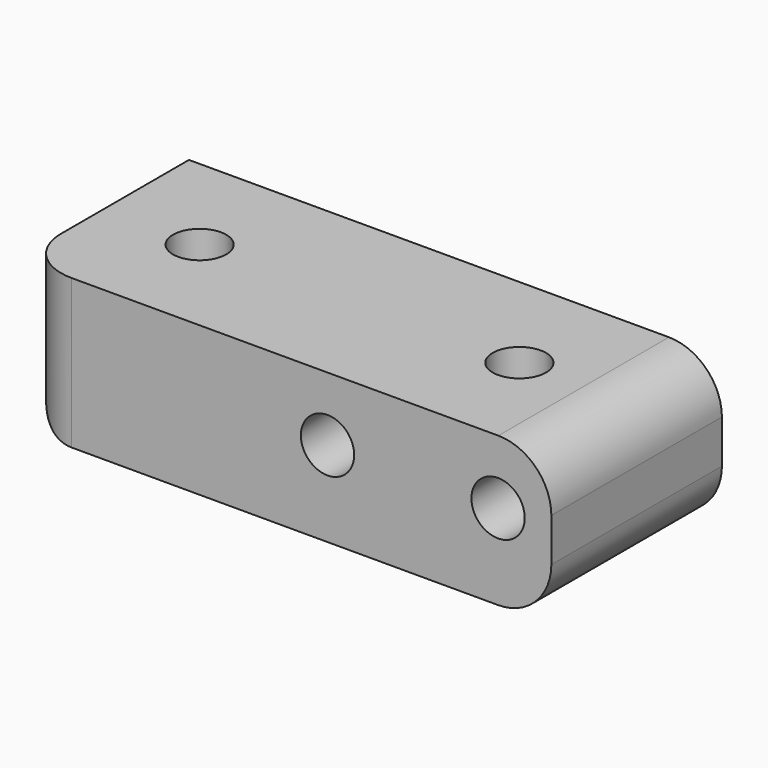
from build123d import *

# Parameters (mm, degrees)
F0_W        = 20
F0_H        = 14
F1_DEPTH    = 25
F3_D        = 5
F5_D        = 5
F6_T1_DEPTH = 44.999500005
F7_T1_DEPTH = 34.0317226184


# Not quite as in the source:
# - a fillet or chamfer that OpenCascade refuses, or shapes differently, is made with other operations: its cross-section is extruded or revolved along the edge and cut away or added


with BuildPart() as f1:
    # F0 (on Right) → F1 (new body, symmetric)
    with BuildSketch(Plane.YZ):
        Rectangle(F0_W, F0_H)
    extrude(amount=F1_DEPTH, both=True)

    # F3 (through all)
    with Locations(Plane.XZ.offset(10)):
        with Locations((4, 1), (20, 1)):
            Hole(F3_D / 2)

    # F5 (through all)
    with Locations(Plane.XY.offset(7)):
        with Locations((-16, 0), (14, 0)):
            Hole(F5_D / 2)

    # F6: fillet of radius 5 on 3 edges, made by hand

    # F6_s2 → F6_t1 (cut)
    with BuildSketch(Plane.XZ.offset(-22.4997500025)):
        with BuildLine():
            ThreePointArc((25.0001, 2.0001), (23.5356339059, 5.5356339059), (20.0001, 7.0001))
            Line((20.0001, 7.0001), (20.0001, 7.1001))
            ThreePointArc((20.0001, 7.1001), (22.50005, 7.1), (25, 7.1))
            Line((25, 7.1), (25.1, 7))
            ThreePointArc((25.1, 7), (25.1, 4.50005), (25.1001, 2.0001))
            Line((25.1001, 2.0001), (25.0001, 2.0001))
        make_face()
        with BuildLine():
            ThreePointArc((-20.0001, -7.0001), (-23.5356339059, -5.5356339059), (-25.0001, -2.0001))
            Line((-25.0001, -2.0001), (-25.1001, -2.0001))
            ThreePointArc((-25.1001, -2.0001), (-25.1, -4.50005), (-25.1, -7))
            Line((-25.1, -7), (-25, -7.1))
            ThreePointArc((-25, -7.1), (-22.50005, -7.1), (-20.0001, -7.1001))
            Line((-20.0001, -7.1001), (-20.0001, -7.0001))
        make_face()
        with BuildLine():
            ThreePointArc((20.0001, -7.0001), (23.5356339059, -5.5356339059), (25.0001, -2.0001))
            Line((25.0001, -2.0001), (25.1001, -2.0001))
            ThreePointArc((25.1001, -2.0001), (25.1, -4.50005), (25.1, -7))
            Line((25.1, -7), (25, -7.1))
            ThreePointArc((25, -7.1), (22.50005, -7.1), (20.0001, -7.1001))
            Line((20.0001, -7.1001), (20.0001, -7.0001))
        make_face()
    extrude(amount=F6_T1_DEPTH, mode=Mode.SUBTRACT)

    # F7: fillet of radius 5 on 1 edges, made by hand

    # F7_s2 → F7_t1 (cut)
    with BuildSketch(Plane.XY.offset(-14.5317226184)):
        with BuildLine():
            ThreePointArc((-20, -10), (-23.5355339059, -8.5355339059), (-25, -5))
            Line((-25, -5), (-25, -10))
            Line((-25, -10), (-20, -10))
        make_face()
    extrude(amount=F7_T1_DEPTH, mode=Mode.SUBTRACT)


solid = f1.part
